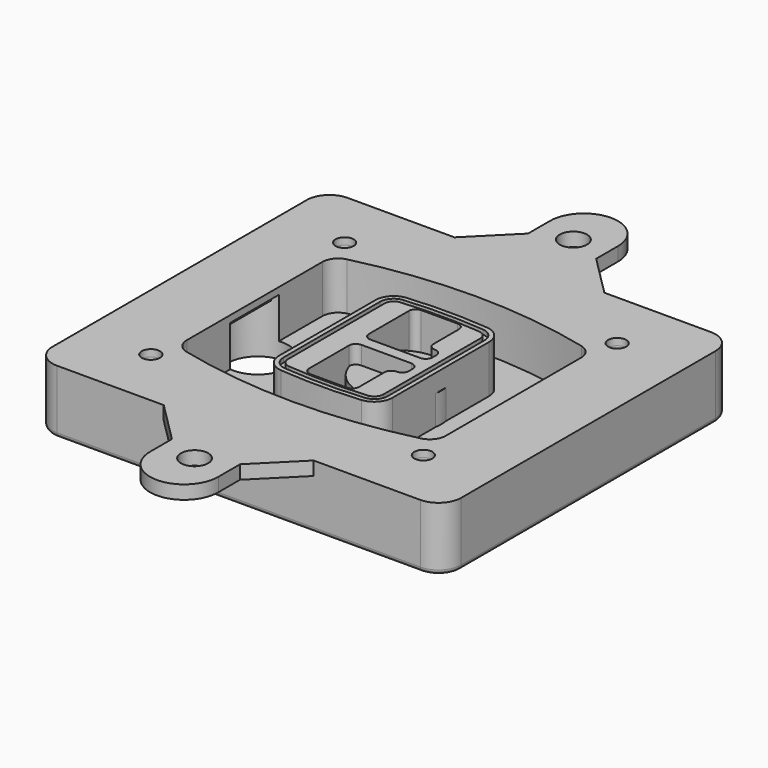
from build123d import *

# Parameters (mm, degrees)
F0_R      = 4
F1_DEPTH  = 25
F2_DEPTH  = 3
F3_DEPTH  = 18
F5_DEPTH  = 21
F6_DEPTH  = 2
F8_DEPTH  = 20
F9_DEPTH  = 16
F10_DEPTH = 25
F7_R      = 6
F7_R_2    = 4
F11_DEPTH = 6
F13_DEPTH = 9
F15_R     = 2
F16_R     = 4
F16_R_2   = 6
F17_DEPTH = 3


# Not quite as in the source:
# - a feature of the source that left no trace in its solid (it failed there, or was rolled back) is left out
# - a feature names something its author has since deleted; it is built from what else it names


with BuildPart() as f1:
    # F0 (on Top) → F1 (new body)
    with BuildSketch(Plane.XY):
        with BuildLine():
            ThreePointArc((-90, -70), (-87.0710678119, -77.0710678119), (-80, -80))
            Line((-80, -80), (80, -80))
            ThreePointArc((80, -80), (87.0710678119, -77.0710678119), (90, -70))
            Line((90, -70), (90, 70))
            ThreePointArc((90, 70), (87.0710678119, 77.0710678119), (80, 80))
            Line((80, 80), (-80, 80))
            ThreePointArc((-80, 80), (-87.0710678119, 77.0710678119), (-90, 70))
            Line((-90, 70), (-90, -70))
        make_face()
        with Locations((-60, -53.3333333333)):
            Circle(F0_R, mode=Mode.SUBTRACT)
        with Locations((60, -53.3333333333)):
            Circle(F0_R, mode=Mode.SUBTRACT)
        with Locations((-60, 53.3333333333)):
            Circle(F0_R, mode=Mode.SUBTRACT)
        with BuildLine():
            ThreePointArc((-64, 37.2990447398), (-61.0143011354, 45.9411029726), (-53.3306899286, 50.8970778549))
            ThreePointArc((-53.3306899286, 50.8970778549), (0, 57.3333333333), (53.3306899286, 50.8970778549))
            ThreePointArc((53.3306899286, 50.8970778549), (61.0143011354, 45.9411029726), (64, 37.2990447398))
            Line((64, 37.2990447398), (64, -37.2990447398))
            ThreePointArc((64, -37.2990447398), (61.0143011354, -45.9411029726), (53.3306899286, -50.8970778549))
            ThreePointArc((53.3306899286, -50.8970778549), (0, -57.3333333333), (-53.3306899286, -50.8970778549))
            ThreePointArc((-53.3306899286, -50.8970778549), (-61.0143011354, -45.9411029726), (-64, -37.2990447398))
            Line((-64, -37.2990447398), (-64, 37.2990447398))
        make_face(mode=Mode.SUBTRACT)
        with Locations((60, 53.3333333333)):
            Circle(F0_R, mode=Mode.SUBTRACT)
        with BuildLine():
            ThreePointArc((53.3306899286, 50.8970778549), (0, 57.3333333333), (-53.3306899286, 50.8970778549))
            ThreePointArc((-53.3306899286, 50.8970778549), (-61.0143011354, 45.9411029726), (-64, 37.2990447398))
            Line((-64, 37.2990447398), (-64, -37.2990447398))
            ThreePointArc((-64, -37.2990447398), (-61.0143011354, -45.9411029726), (-53.3306899286, -50.8970778549))
            ThreePointArc((-53.3306899286, -50.8970778549), (0, -57.3333333333), (53.3306899286, -50.8970778549))
            ThreePointArc((53.3306899286, -50.8970778549), (61.0143011354, -45.9411029726), (64, -37.2990447398))
            Line((64, -37.2990447398), (64, 37.2990447398))
            ThreePointArc((64, 37.2990447398), (61.0143011354, 45.9411029726), (53.3306899286, 50.8970778549))
        make_face()
        with BuildLine():
            Line((-60, -37.2990447398), (-60, 37.2990447398))
            ThreePointArc((-60, 37.2990447398), (-57.8673579538, 43.4719434775), (-52.3790642347, 47.0119255363))
            ThreePointArc((-52.3790642347, 47.0119255363), (0, 53.3333333333), (52.3790642347, 47.0119255363))
            ThreePointArc((52.3790642347, 47.0119255363), (57.8673579538, 43.4719434775), (60, 37.2990447398))
            Line((60, 37.2990447398), (60, -37.2990447398))
            ThreePointArc((60, -37.2990447398), (57.8673579538, -43.4719434775), (52.3790642347, -47.0119255363))
            ThreePointArc((52.3790642347, -47.0119255363), (0, -53.3333333333), (-52.3790642347, -47.0119255363))
            ThreePointArc((-52.3790642347, -47.0119255363), (-57.8673579538, -43.4719434775), (-60, -37.2990447398))
        make_face(mode=Mode.SUBTRACT)
        with BuildLine():
            ThreePointArc((-52.3790642347, 47.0119255363), (-57.8673579538, 43.4719434775), (-60, 37.2990447398))
            Line((-60, 37.2990447398), (-60, -37.2990447398))
            ThreePointArc((-60, -37.2990447398), (-57.8673579538, -43.4719434775), (-52.3790642347, -47.0119255363))
            ThreePointArc((-52.3790642347, -47.0119255363), (0, -53.3333333333), (52.3790642347, -47.0119255363))
            ThreePointArc((52.3790642347, -47.0119255363), (57.8673579538, -43.4719434775), (60, -37.2990447398))
            Line((60, -37.2990447398), (60, 37.2990447398))
            ThreePointArc((60, 37.2990447398), (57.8673579538, 43.4719434775), (52.3790642347, 47.0119255363))
            ThreePointArc((52.3790642347, 47.0119255363), (0, 53.3333333333), (-52.3790642347, 47.0119255363))
        make_face()
        with BuildLine():
            ThreePointArc((51.6653449643, 44.0980612973), (55.5071505677, 41.6200738562), (57, 37.2990447398))
            Line((57, 37.2990447398), (57, -37.2990447398))
            ThreePointArc((57, -37.2990447398), (55.5071505677, -41.6200738562), (51.6653449643, -44.0980612973))
            ThreePointArc((51.6653449643, -44.0980612973), (0, -50.3333333333), (-51.6653449643, -44.0980612973))
            ThreePointArc((-51.6653449643, -44.0980612973), (-55.5071505677, -41.6200738562), (-57, -37.2990447398))
            Line((-57, -37.2990447398), (-57, 37.2990447398))
            ThreePointArc((-57, 37.2990447398), (-55.5071505677, 41.6200738562), (-51.6653449643, 44.0980612973))
            ThreePointArc((-51.6653449643, 44.0980612973), (0, 50.3333333333), (51.6653449643, 44.0980612973))
        make_face(mode=Mode.SUBTRACT)
        with BuildLine():
            Line((57, -37.2990447398), (57, 37.2990447398))
            ThreePointArc((57, 37.2990447398), (55.5071505677, 41.6200738562), (51.6653449643, 44.0980612973))
            ThreePointArc((51.6653449643, 44.0980612973), (0, 50.3333333333), (-51.6653449643, 44.0980612973))
            ThreePointArc((-51.6653449643, 44.0980612973), (-55.5071505677, 41.6200738562), (-57, 37.2990447398))
            Line((-57, 37.2990447398), (-57, -37.2990447398))
            ThreePointArc((-57, -37.2990447398), (-55.5071505677, -41.6200738562), (-51.6653449643, -44.0980612973))
            ThreePointArc((-51.6653449643, -44.0980612973), (0, -50.3333333333), (51.6653449643, -44.0980612973))
            ThreePointArc((51.6653449643, -44.0980612973), (55.5071505677, -41.6200738562), (57, -37.2990447398))
        make_face()
    extrude(amount=-F1_DEPTH)

    # F0 (on Top) → F2 (join)
    with BuildSketch(Plane.XY):
        with BuildLine():
            ThreePointArc((-52.3790642347, 47.0119255363), (-57.8673579538, 43.4719434775), (-60, 37.2990447398))
            Line((-60, 37.2990447398), (-60, -37.2990447398))
            ThreePointArc((-60, -37.2990447398), (-57.8673579538, -43.4719434775), (-52.3790642347, -47.0119255363))
            ThreePointArc((-52.3790642347, -47.0119255363), (0, -53.3333333333), (52.3790642347, -47.0119255363))
            ThreePointArc((52.3790642347, -47.0119255363), (57.8673579538, -43.4719434775), (60, -37.2990447398))
            Line((60, -37.2990447398), (60, 37.2990447398))
            ThreePointArc((60, 37.2990447398), (57.8673579538, 43.4719434775), (52.3790642347, 47.0119255363))
            ThreePointArc((52.3790642347, 47.0119255363), (0, 53.3333333333), (-52.3790642347, 47.0119255363))
        make_face()
        with BuildLine():
            ThreePointArc((51.6653449643, 44.0980612973), (55.5071505677, 41.6200738562), (57, 37.2990447398))
            Line((57, 37.2990447398), (57, -37.2990447398))
            ThreePointArc((57, -37.2990447398), (55.5071505677, -41.6200738562), (51.6653449643, -44.0980612973))
            ThreePointArc((51.6653449643, -44.0980612973), (0, -50.3333333333), (-51.6653449643, -44.0980612973))
            ThreePointArc((-51.6653449643, -44.0980612973), (-55.5071505677, -41.6200738562), (-57, -37.2990447398))
            Line((-57, -37.2990447398), (-57, 37.2990447398))
            ThreePointArc((-57, 37.2990447398), (-55.5071505677, 41.6200738562), (-51.6653449643, 44.0980612973))
            ThreePointArc((-51.6653449643, 44.0980612973), (0, 50.3333333333), (51.6653449643, 44.0980612973))
        make_face(mode=Mode.SUBTRACT)
    extrude(amount=F2_DEPTH)

    # F0 (on Top) → F3 (cut)
    with BuildSketch(Plane.XY):
        with BuildLine():
            Line((57, -37.2990447398), (57, 37.2990447398))
            ThreePointArc((57, 37.2990447398), (55.5071505677, 41.6200738562), (51.6653449643, 44.0980612973))
            ThreePointArc((51.6653449643, 44.0980612973), (0, 50.3333333333), (-51.6653449643, 44.0980612973))
            ThreePointArc((-51.6653449643, 44.0980612973), (-55.5071505677, 41.6200738562), (-57, 37.2990447398))
            Line((-57, 37.2990447398), (-57, -37.2990447398))
            ThreePointArc((-57, -37.2990447398), (-55.5071505677, -41.6200738562), (-51.6653449643, -44.0980612973))
            ThreePointArc((-51.6653449643, -44.0980612973), (0, -50.3333333333), (51.6653449643, -44.0980612973))
            ThreePointArc((51.6653449643, -44.0980612973), (55.5071505677, -41.6200738562), (57, -37.2990447398))
        make_face()
    extrude(amount=-F3_DEPTH, mode=Mode.SUBTRACT)

    # F4 (on face) → F5 (join, through all)
    with BuildSketch(Plane.XY.offset(3)):
        with BuildLine():
            ThreePointArc((-25, -26.587695628), (-22.8992979869, -31.9912392117), (-17.7004291845, -34.5569740744))
            ThreePointArc((-17.7004291845, -34.5569740744), (0, -35.3333333333), (17.7004291845, -34.5569740744))
            ThreePointArc((17.7004291845, -34.5569740744), (22.8992979869, -31.9912392117), (25, -26.587695628))
            Line((25, -26.587695628), (25, 26.587695628))
            ThreePointArc((25, 26.587695628), (22.8992979869, 31.9912392117), (17.7004291845, 34.5569740744))
            ThreePointArc((17.7004291845, 34.5569740744), (0, 35.3333333333), (-17.7004291845, 34.5569740744))
            ThreePointArc((-17.7004291845, 34.5569740744), (-22.8992979869, 31.9912392117), (-25, 26.587695628))
            Line((-25, 26.587695628), (-25, -26.587695628))
        make_face()
        with BuildLine():
            ThreePointArc((17.5253218884, 32.5646544628), (21.4244734902, 30.6403533158), (23, 26.587695628))
            Line((23, 26.587695628), (23, -26.587695628))
            ThreePointArc((23, -26.587695628), (21.4244734902, -30.6403533158), (17.5253218884, -32.5646544628))
            ThreePointArc((17.5253218884, -32.5646544628), (0, -33.3333333333), (-17.5253218884, -32.5646544628))
            ThreePointArc((-17.5253218884, -32.5646544628), (-21.4244734902, -30.6403533158), (-23, -26.587695628))
            Line((-23, -26.587695628), (-23, 26.587695628))
            ThreePointArc((-23, 26.587695628), (-21.4244734902, 30.6403533158), (-17.5253218884, 32.5646544628))
            ThreePointArc((-17.5253218884, 32.5646544628), (0, 33.3333333333), (17.5253218884, 32.5646544628))
        make_face(mode=Mode.SUBTRACT)
        with BuildLine():
            Line((23, -26.587695628), (23, 26.587695628))
            ThreePointArc((23, 26.587695628), (21.4244734902, 30.6403533158), (17.5253218884, 32.5646544628))
            ThreePointArc((17.5253218884, 32.5646544628), (0, 33.3333333333), (-17.5253218884, 32.5646544628))
            ThreePointArc((-17.5253218884, 32.5646544628), (-21.4244734902, 30.6403533158), (-23, 26.587695628))
            Line((-23, 26.587695628), (-23, -26.587695628))
            ThreePointArc((-23, -26.587695628), (-21.4244734902, -30.6403533158), (-17.5253218884, -32.5646544628))
            ThreePointArc((-17.5253218884, -32.5646544628), (0, -33.3333333333), (17.5253218884, -32.5646544628))
            ThreePointArc((17.5253218884, -32.5646544628), (21.4244734902, -30.6403533158), (23, -26.587695628))
        make_face()
        with BuildLine():
            ThreePointArc((17.3502145923, 30.5723348512), (19.9496489934, 29.2894674198), (21, 26.587695628))
            Line((21, 26.587695628), (21, -26.587695628))
            ThreePointArc((21, -26.587695628), (19.9496489934, -29.2894674198), (17.3502145923, -30.5723348512))
            ThreePointArc((17.3502145923, -30.5723348512), (0, -31.3333333333), (-17.3502145923, -30.5723348512))
            ThreePointArc((-17.3502145923, -30.5723348512), (-19.9496489934, -29.2894674198), (-21, -26.587695628))
            Line((-21, -26.587695628), (-21, 26.587695628))
            ThreePointArc((-21, 26.587695628), (-19.9496489934, 29.2894674198), (-17.3502145923, 30.5723348512))
            ThreePointArc((-17.3502145923, 30.5723348512), (0, 31.3333333333), (17.3502145923, 30.5723348512))
        make_face(mode=Mode.SUBTRACT)
        with BuildLine():
            Line((21, -26.587695628), (21, 26.587695628))
            ThreePointArc((21, 26.587695628), (19.9496489934, 29.2894674198), (17.3502145923, 30.5723348512))
            ThreePointArc((17.3502145923, 30.5723348512), (0, 31.3333333333), (-17.3502145923, 30.5723348512))
            ThreePointArc((-17.3502145923, 30.5723348512), (-19.9496489934, 29.2894674198), (-21, 26.587695628))
            Line((-21, 26.587695628), (-21, -26.587695628))
            ThreePointArc((-21, -26.587695628), (-19.9496489934, -29.2894674198), (-17.3502145923, -30.5723348512))
            ThreePointArc((-17.3502145923, -30.5723348512), (0, -31.3333333333), (17.3502145923, -30.5723348512))
            ThreePointArc((17.3502145923, -30.5723348512), (19.9496489934, -29.2894674198), (21, -26.587695628))
        make_face()
        with BuildLine():
            Line((-8, -2.5), (14, -2.5))
            ThreePointArc((14, -2.5), (16.1213203436, -3.3786796564), (17, -5.5))
            Line((17, -5.5), (17, -7.5))
            ThreePointArc((17, -7.5), (16.1213203436, -9.6213203436), (14, -10.5))
            ThreePointArc((14, -10.5), (11.8786796564, -11.3786796564), (11, -13.5))
            Line((11, -13.5), (11, -27.5))
            ThreePointArc((11, -27.5), (10.1213203436, -29.6213203436), (8, -30.5))
            Line((8, -30.5), (-8, -30.5))
            ThreePointArc((-8, -30.5), (-10.1213203436, -29.6213203436), (-11, -27.5))
            Line((-11, -27.5), (-11, -5.5))
            ThreePointArc((-11, -5.5), (-10.1213203436, -3.3786796564), (-8, -2.5))
        make_face(mode=Mode.SUBTRACT)
        with BuildLine():
            ThreePointArc((-8, 2.5), (-10.1213203436, 3.3786796564), (-11, 5.5))
            Line((-11, 5.5), (-11, 27.5))
            ThreePointArc((-11, 27.5), (-10.1213203436, 29.6213203436), (-8, 30.5))
            Line((-8, 30.5), (8, 30.5))
            ThreePointArc((8, 30.5), (10.1213203436, 29.6213203436), (11, 27.5))
            Line((11, 27.5), (11, 13.5))
            ThreePointArc((11, 13.5), (11.8786796564, 11.3786796564), (14, 10.5))
            ThreePointArc((14, 10.5), (16.1213203436, 9.6213203436), (17, 7.5))
            Line((17, 7.5), (17, 5.5))
            ThreePointArc((17, 5.5), (16.1213203436, 3.3786796564), (14, 2.5))
            Line((14, 2.5), (-8, 2.5))
        make_face(mode=Mode.SUBTRACT)
    extrude(amount=-F5_DEPTH)

    # F4 (on face) → F6 (cut)
    with BuildSketch(Plane.XY.offset(3)):
        with BuildLine():
            Line((23, -26.587695628), (23, 26.587695628))
            ThreePointArc((23, 26.587695628), (21.4244734902, 30.6403533158), (17.5253218884, 32.5646544628))
            ThreePointArc((17.5253218884, 32.5646544628), (0, 33.3333333333), (-17.5253218884, 32.5646544628))
            ThreePointArc((-17.5253218884, 32.5646544628), (-21.4244734902, 30.6403533158), (-23, 26.587695628))
            Line((-23, 26.587695628), (-23, -26.587695628))
            ThreePointArc((-23, -26.587695628), (-21.4244734902, -30.6403533158), (-17.5253218884, -32.5646544628))
            ThreePointArc((-17.5253218884, -32.5646544628), (0, -33.3333333333), (17.5253218884, -32.5646544628))
            ThreePointArc((17.5253218884, -32.5646544628), (21.4244734902, -30.6403533158), (23, -26.587695628))
        make_face()
        with BuildLine():
            ThreePointArc((17.3502145923, 30.5723348512), (19.9496489934, 29.2894674198), (21, 26.587695628))
            Line((21, 26.587695628), (21, -26.587695628))
            ThreePointArc((21, -26.587695628), (19.9496489934, -29.2894674198), (17.3502145923, -30.5723348512))
            ThreePointArc((17.3502145923, -30.5723348512), (0, -31.3333333333), (-17.3502145923, -30.5723348512))
            ThreePointArc((-17.3502145923, -30.5723348512), (-19.9496489934, -29.2894674198), (-21, -26.587695628))
            Line((-21, -26.587695628), (-21, 26.587695628))
            ThreePointArc((-21, 26.587695628), (-19.9496489934, 29.2894674198), (-17.3502145923, 30.5723348512))
            ThreePointArc((-17.3502145923, 30.5723348512), (0, 31.3333333333), (17.3502145923, 30.5723348512))
        make_face(mode=Mode.SUBTRACT)
    extrude(amount=-F6_DEPTH, mode=Mode.SUBTRACT)

    # F7 (on face) → F8 (join)
    with BuildSketch(Plane(origin=(0, 0, -25), x_dir=(1, 0, 0), z_dir=(0, 0, -1))):
        with BuildLine():
            ThreePointArc((-6.71157564, 0), (6.7567035675, 13.4682792075), (20.224982775, 0))
            Line((20.224982775, 0), (25.224982775, 0))
            ThreePointArc((25.224982775, 0), (6.7567035675, 18.4682792075), (-11.71157564, 0))
            Line((-11.71157564, 0), (-6.71157564, 0))
        make_face()
        with BuildLine():
            Line((-6.71157564, 0), (20.224982775, 0))
            ThreePointArc((20.224982775, 0), (6.7567035675, 13.4682792075), (-6.71157564, 0))
        make_face()
        with BuildLine():
            ThreePointArc((-6.71157564, 0), (6.7567035675, -13.4682792075), (20.224982775, 0))
            Line((20.224982775, 0), (-6.71157564, 0))
        make_face()
        with BuildLine():
            Line((25.224982775, 0), (20.224982775, 0))
            ThreePointArc((20.224982775, 0), (6.7567035675, -13.4682792075), (-6.71157564, 0))
            Line((-6.71157564, 0), (-11.71157564, 0))
            ThreePointArc((-11.71157564, 0), (6.7567035675, -18.4682792075), (25.224982775, 0))
        make_face()
    extrude(amount=-F8_DEPTH)

    # F7 (on face) → F9 (cut)
    with BuildSketch(Plane(origin=(0, 0, -25), x_dir=(1, 0, 0), z_dir=(0, 0, -1))):
        with BuildLine():
            Line((-6.71157564, 0), (20.224982775, 0))
            ThreePointArc((20.224982775, 0), (6.7567035675, 13.4682792075), (-6.71157564, 0))
        make_face()
        with BuildLine():
            ThreePointArc((-6.71157564, 0), (6.7567035675, -13.4682792075), (20.224982775, 0))
            Line((20.224982775, 0), (-6.71157564, 0))
        make_face()
    extrude(amount=-F9_DEPTH, mode=Mode.SUBTRACT)

    # F7 (on face) → F10 (cut)
    with BuildSketch(Plane(origin=(0, 0, -25), x_dir=(1, 0, 0), z_dir=(0, 0, -1))):
        with BuildLine():
            Line((-69.0318229325, 0), (-42.0952645175, 0))
            ThreePointArc((-42.0952645175, 0), (-55.563543725, 13.4682792075), (-69.0318229325, 0))
        make_face()
        with BuildLine():
            ThreePointArc((-69.0318229325, 0), (-55.563543725, -13.4682792075), (-42.0952645175, 0))
            Line((-42.0952645175, 0), (-69.0318229325, 0))
        make_face()
    extrude(amount=-F10_DEPTH, mode=Mode.SUBTRACT)

    # F7 (on face) → F11 (cut)
    with BuildSketch(Plane(origin=(0, 0, -25), x_dir=(1, 0, 0), z_dir=(0, 0, -1))):
        with Locations((60, -53.3333333333)):
            Circle(F7_R)
        with Locations((60, -53.3333333333)):
            Circle(F7_R_2, mode=Mode.SUBTRACT)
        with Locations((-60, -53.3333333333)):
            Circle(F7_R)
        with Locations((-60, -53.3333333333)):
            Circle(F7_R_2, mode=Mode.SUBTRACT)
        with Locations((-60, 53.3333333333)):
            Circle(F7_R)
        with Locations((-60, 53.3333333333)):
            Circle(F7_R_2, mode=Mode.SUBTRACT)
        with Locations((60, 53.3333333333)):
            Circle(F7_R)
        with Locations((60, 53.3333333333)):
            Circle(F7_R_2, mode=Mode.SUBTRACT)
    extrude(amount=-F11_DEPTH, mode=Mode.SUBTRACT)

    # F12 (on face) → F13 (cut, through all)
    with BuildSketch(Plane(origin=(0, 0, -9), x_dir=(1, 0, 0), z_dir=(0, 0, -1))):
        with BuildLine():
            ThreePointArc((20.224982775, 0), (20.1663399806, 1.2554664788), (19.9909222755, 2.5))
            Line((19.9909222755, 2.5), (14, 2.5))
            ThreePointArc((14, 2.5), (16.1213203436, 3.3786796564), (17, 5.5))
            Line((17, 5.5), (17, 7.5))
            ThreePointArc((17, 7.5), (16.1213203436, 9.6213203436), (14, 10.5))
            ThreePointArc((14, 10.5), (12.1627255951, 11.1284134507), (11.0951631559, 12.750384826))
            ThreePointArc((11.0951631559, 12.750384826), (11.0476113807, 12.7664660322), (11, 12.7823698976))
            Line((11, 12.7823698976), (11, -12.7823698976))
            ThreePointArc((11, -12.7823698976), (11.0476113807, -12.7664660322), (11.0951631559, -12.750384826))
            ThreePointArc((11.0951631559, -12.750384826), (12.1627255951, -11.1284134507), (14, -10.5))
            ThreePointArc((14, -10.5), (16.1213203436, -9.6213203436), (17, -7.5))
            Line((17, -7.5), (17, -5.5))
            ThreePointArc((17, -5.5), (16.1213203436, -3.3786796564), (14, -2.5))
            Line((14, -2.5), (19.9909222755, -2.5))
            ThreePointArc((19.9909222755, -2.5), (20.1663399806, -1.2554664788), (20.224982775, 0))
        make_face()
    extrude(amount=F13_DEPTH, mode=Mode.SUBTRACT)

    # F15
    f15_edges = [f1.edges().sort_by_distance(p)[0] for p in [
        (0, -80, -25),
        (-87.071068, -77.071068, -25),
        (-90, 0, -25),
        (-87.071068, 77.071068, -25),
        (87.071068, -77.071068, -25),
        (0, 80, -25),
        (90, 0, -25),
        (87.071068, 77.071068, -25),
    ]]
    fillet(f15_edges, radius=F15_R)

    # F16 (on face) → F17 (join, symmetric)
    with BuildSketch(Plane.XY):
        with BuildLine():
            Line((90, -70), (90, 70))
            ThreePointArc((90, 70), (87.0710678119, 77.0710678119), (80, 80))
            Line((80, 80), (33.0211562589, 80))
            Line((33.0211562589, 80), (-32.9788437411, 80))
            Line((-32.9788437411, 80), (-80, 80))
            ThreePointArc((-80, 80), (-87.0710678119, 77.0710678119), (-90, 70))
            Line((-90, 70), (-90, -70))
            ThreePointArc((-90, -70), (-87.0710678119, -77.0710678119), (-80, -80))
            Line((-80, -80), (-32.9788437411, -80))
            Line((-32.9788437411, -80), (33.0211562589, -80))
            Line((33.0211562589, -80), (80, -80))
            ThreePointArc((80, -80), (87.0710678119, -77.0710678119), (90, -70))
        make_face()
        with Locations((-60, -53.3333333333)):
            Circle(F16_R, mode=Mode.SUBTRACT)
        with Locations((60, -53.3333333333)):
            Circle(F16_R, mode=Mode.SUBTRACT)
        with Locations((-60, 53.3333333333)):
            Circle(F16_R, mode=Mode.SUBTRACT)
        with BuildLine():
            Line((-60, -37.2990447398), (-60, 37.2990447398))
            ThreePointArc((-60, 37.2990447398), (-57.8673579538, 43.4719434775), (-52.3790642347, 47.0119255363))
            ThreePointArc((-52.3790642347, 47.0119255363), (0, 53.3333333333), (52.3790642347, 47.0119255363))
            ThreePointArc((52.3790642347, 47.0119255363), (57.8673579538, 43.4719434775), (60, 37.2990447398))
            Line((60, 37.2990447398), (60, -37.2990447398))
            ThreePointArc((60, -37.2990447398), (57.8673579538, -43.4719434775), (52.3790642347, -47.0119255363))
            ThreePointArc((52.3790642347, -47.0119255363), (0, -53.3333333333), (-52.3790642347, -47.0119255363))
            ThreePointArc((-52.3790642347, -47.0119255363), (-57.8673579538, -43.4719434775), (-60, -37.2990447398))
        make_face(mode=Mode.SUBTRACT)
        with Locations((60, 53.3333333333)):
            Circle(F16_R, mode=Mode.SUBTRACT)
        with BuildLine():
            Line((-32.9788437411, 80), (33.0211562589, 80))
            Line((33.0211562589, 80), (15.0211562589, 98))
            Line((15.0211562589, 98), (15.0211562589, 110))
            ThreePointArc((15.0211562589, 110), (0.0211562589, 125), (-14.9788437411, 110))
            Line((-14.9788437411, 110), (-14.9788437411, 98))
            Line((-14.9788437411, 98), (-32.9788437411, 80))
        make_face()
        with Locations((0, 104.25)):
            Circle(F16_R_2, mode=Mode.SUBTRACT)
        with BuildLine():
            Line((15.0211562589, -98), (33.0211562589, -80))
            Line((33.0211562589, -80), (-32.9788437411, -80))
            Line((-32.9788437411, -80), (-14.9788437411, -98))
            Line((-14.9788437411, -98), (-14.9788437411, -110))
            ThreePointArc((-14.9788437411, -110), (0.0211562589, -125), (15.0211562589, -110))
            Line((15.0211562589, -110), (15.0211562589, -98))
        make_face()
        with Locations((0, -104.25)):
            Circle(F16_R_2, mode=Mode.SUBTRACT)
    extrude(amount=F17_DEPTH, both=True)


solid = f1.part
